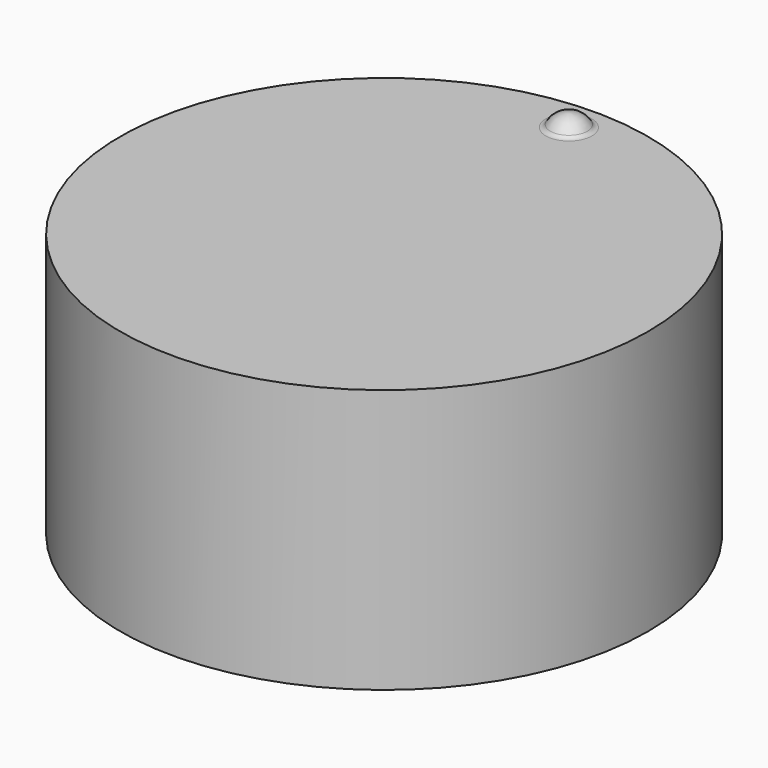
from build123d import *

# Parameters (mm, degrees)
F0_R     = 10
F0_R_2   = 2.5
F0_R_3   = 0.75
F1_DEPTH = 10
F2_DEPTH = 8
F3_DEPTH = 10.5
F5_R     = 0.2


# Not quite as in the source:
# - a fillet or chamfer that OpenCascade refuses, or shapes differently, is made with other operations: its cross-section is extruded or revolved along the edge and cut away or added


with BuildPart() as f1:
    # F0 (on Top) → F1 (new body)
    with BuildSketch(Plane.XY):
        Circle(F0_R)
        Circle(F0_R_2, mode=Mode.SUBTRACT)
        with Locations((0, 8.75)):
            Circle(F0_R_3, mode=Mode.SUBTRACT)
        with Locations((0, 8.75)):
            Circle(F0_R_3)
        Circle(F0_R_2)
    extrude(amount=F1_DEPTH)

    # F0 (on Top) → F2 (cut)
    with BuildSketch(Plane.XY):
        Circle(F0_R_2)
    extrude(amount=F2_DEPTH, mode=Mode.SUBTRACT)

    # F0 (on Top) → F3 (join)
    with BuildSketch(Plane.XY):
        with Locations((0, 8.75)):
            Circle(F0_R_3)
    extrude(amount=F3_DEPTH)

    # F4: fillet of radius 0.798 on 1 edges, made by hand

    # F4_s1 → F4_t2 (revolve, cut)
    with BuildSketch(Plane.XZ.offset(-8.75)):
        with BuildLine():
            ThreePointArc((0.75, 10), (0.4563840077, 10.3632896491), (0.0097297791, 10.5))
            Line((0.0097297791, 10.5), (0.75, 10.5))
            Line((0.75, 10.5), (0.75, 10))
        make_face()
    revolve(axis=Axis((0, 8.75, 10.5), (0, 0, 1)), mode=Mode.SUBTRACT)

    # F5
    f5_edges = [f1.edges().sort_by_distance(p)[0] for p in [
        (-0.75, 8.75, 10),
    ]]
    fillet(f5_edges, radius=F5_R)


solid = f1.part
